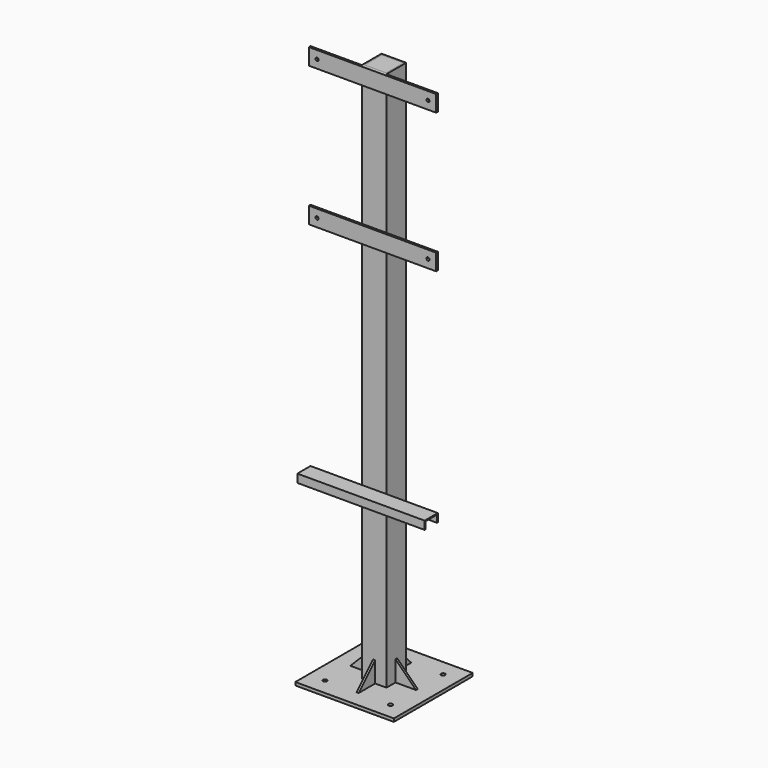
from build123d import *

# Parameters (mm, degrees)
F0_W      = 76.2
F0_H      = 76.2
F0_W_2    = 66.675
F0_H_2    = 66.675
F1_DEPTH  = 2133.6
F2_W      = 66.675
F2_H      = 66.675
F4_DEPTH  = 4.7625
F6_DEPTH  = 457.2
F8_W      = 304.8
F8_H      = 304.8
F8_R      = 6.35
F9_DEPTH  = 6.35
F12_DEPTH = 3.175
F13_DEPTH = 3.175
F15_DEPTH = 3.175
F16_DEPTH = 3.175
F17_DEPTH = 3.175
F5_W      = 158.75
F5_H      = 50.8105754852
F5_R      = 4.7625
F5_W_2    = 76.2
F5_H_2    = 50.8
F18_DEPTH = 6.35
F19_W     = 158.75
F19_H     = 25.4
F19_W_2   = 76.2
F20_DEPTH = 50.8
F21_W     = 44.45
F21_H     = 22.225
F22_DEPTH = 508


# Not quite as in the source:
# - a feature names something its author has since deleted; it is built from what else it names


with BuildPart() as f1:
    # F0 (on Top) → F1 (new body)
    with BuildSketch(Plane.XY):
        with Locations((-0.0228539575, -0.3835560492)):
            Rectangle(F0_W, F0_H)
        with Locations((-0.0228539575, -0.3835560492)):
            Rectangle(F0_W_2, F0_H_2, mode=Mode.SUBTRACT)
    extrude(amount=F1_DEPTH)

    # F6 (cut): a face of the model
    f6_faces = [f1.faces().sort_by_distance(p)[0] for p in [
        (-0.0228539575, 36.6388132163, 0),
    ]]
    extrude(f6_faces, amount=-F6_DEPTH, mode=Mode.SUBTRACT)

    # F8 (on offset) → F9 (join)
    with BuildSketch(Plane(origin=(0, 0, 457.2), x_dir=(1, 0, 0), z_dir=(0, 0, -1))):
        with Locations((-0.0228539575, 0.3835560492)):
            Rectangle(F8_W, F8_H)
        with Locations((-101.6228539575, -101.2164439508)):
            Circle(F8_R, mode=Mode.SUBTRACT)
        with Locations((101.5771460425, -101.2164439508)):
            Circle(F8_R, mode=Mode.SUBTRACT)
        with Locations((-101.6228539575, 101.9835560492)):
            Circle(F8_R, mode=Mode.SUBTRACT)
        with Locations((101.5771460425, 101.9835560492)):
            Circle(F8_R, mode=Mode.SUBTRACT)
    extrude(amount=-F9_DEPTH)

    # F8 (on offset) → F12 (join)
    with BuildSketch(Plane(origin=(0, 0, 457.2), x_dir=(1, 0, 0), z_dir=(0, 0, -1))):
        with Locations((-0.0228539575, 0.3835560492)):
            Rectangle(F8_W, F8_H)
        with Locations((-101.6228539575, -101.2164439508)):
            Circle(F8_R, mode=Mode.SUBTRACT)
        with Locations((101.5771460425, -101.2164439508)):
            Circle(F8_R, mode=Mode.SUBTRACT)
        with Locations((-101.6228539575, 101.9835560492)):
            Circle(F8_R, mode=Mode.SUBTRACT)
        with Locations((101.5771460425, 101.9835560492)):
            Circle(F8_R, mode=Mode.SUBTRACT)
    extrude(amount=F12_DEPTH)

    # F11 (on offset) → F13 (join)
    with BuildSketch(Plane.XZ.offset(0.3835560492)):
        Polygon((101.5771460425, 463.55), (38.0771460425, 527.05), (38.0771460425, 463.55), align=None)
        Polygon((-38.1228539575, 463.55), (-38.1228539575, 527.05), (-101.6228539575, 463.55), align=None)
    extrude(amount=-F13_DEPTH)

    # F14 (on Right) → F15 (join)
    with BuildSketch(Plane.YZ):
        Polygon((101.2164439508, 463.55), (37.7164439508, 527.05), (37.7164439508, 463.55), align=None)
        Polygon((-38.4835560492, 463.55), (-38.4835560492, 527.05), (-101.9835560492, 463.55), align=None)
    extrude(amount=F15_DEPTH)

    # F14 (on Right) → F16 (join)
    with BuildSketch(Plane.YZ):
        Polygon((101.2164439508, 463.55), (37.7164439508, 527.05), (37.7164439508, 463.55), align=None)
        Polygon((-38.4835560492, 463.55), (-38.4835560492, 527.05), (-101.9835560492, 463.55), align=None)
    extrude(amount=-F16_DEPTH)

    # F11 (on offset) + F13_face (on face) → F17 (join)
    with BuildSketch(Plane.XZ.offset(0.3835560492)):
        Polygon((101.5771460425, 463.55), (38.0771460425, 527.05), (38.0771460425, 463.55), align=None)
        Polygon((-38.1228539575, 463.55), (-38.1228539575, 527.05), (-101.6228539575, 463.55), align=None)
    with BuildSketch(Plane(origin=(59.2438127092, -0.3835560492, 484.7166666667), x_dir=(1, 0, 0), z_dir=(0, -1, 0))):
        Polygon((42.3333333333, -21.1666666667), (-21.1666666667, 42.3333333333), (-21.1666666667, -21.1666666667), align=None)
    extrude(amount=F17_DEPTH)

    # F5 (on face) → F18 (join)
    with BuildSketch(Plane.XZ.offset(38.4835560492)):
        with Locations((-117.4978539575, 1676.3947122574)):
            Rectangle(F5_W, F5_H)
        with Locations((-171.4728539575, 1676.4)):
            Circle(F5_R, mode=Mode.SUBTRACT)
        with Locations((117.4521460425, 1676.3947122574)):
            Rectangle(F5_W, F5_H)
        with Locations((171.4271460425, 1676.4)):
            Circle(F5_R, mode=Mode.SUBTRACT)
        with Locations((-0.0228539575, 1676.3947122574)):
            Rectangle(F5_W_2, F5_H)
        with Locations((-117.4978539575, 2108.2)):
            Rectangle(F5_W, F5_H_2)
        with Locations((-171.4728539575, 2108.2)):
            Circle(F5_R, mode=Mode.SUBTRACT)
        with Locations((-0.0228539575, 2108.2)):
            Rectangle(F5_W_2, F5_H_2)
        with Locations((117.4521460425, 2108.2)):
            Rectangle(F5_W, F5_H_2)
        with Locations((171.4271460425, 2108.2)):
            Circle(F5_R, mode=Mode.SUBTRACT)
    extrude(amount=F18_DEPTH)

    # F19 (on face) → F20 (join)
    with BuildSketch(Plane.XZ.offset(38.4835560492)):
        with Locations((117.4521460425, 977.9)):
            Rectangle(F19_W, F19_H)
        with Locations((-0.0228539575, 977.9)):
            Rectangle(F19_W_2, F19_H)
        with Locations((-117.4978539575, 977.9)):
            Rectangle(F19_W, F19_H)
    extrude(amount=F20_DEPTH)

    # F21 (on face) → F22 (cut)
    with BuildSketch(Plane.YZ.offset(196.8271460425)):
        with Locations((-63.8835560492, 976.3125)):
            Rectangle(F21_W, F21_H)
    extrude(amount=-F22_DEPTH, mode=Mode.SUBTRACT)


with BuildPart() as f4:
    # F2 (on face) → F4 (new body)
    with BuildSketch(Plane.XY.offset(2133.6)):
        with Locations((-0.0228539575, -0.3835560492)):
            Rectangle(F2_W, F2_H)
    extrude(amount=-F4_DEPTH)


solid = Compound([f1.part, f4.part])
